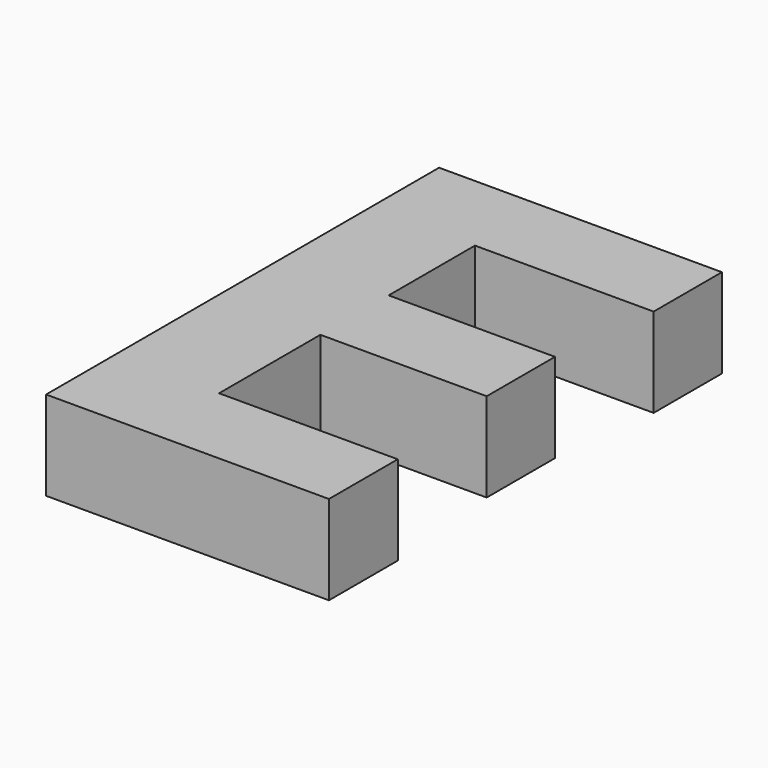
from build123d import *

# Parameters (mm, degrees)
F0_TEXT_SIZE = 77.1269667894
F1_DEPTH     = 10


# Not quite as in the source:
# - Text() gives the source's letters only with a copy of the font that has no kerning and outlines rounded to 1/6400 em; it was checked with that copy


with BuildPart() as f1:
    # F0 (on Top) → F1 (new body)
    with BuildSketch(Plane.XY):
        with Locations((0, 0)):
            Text('E', F0_TEXT_SIZE, font='Open Sans', font_style=FontStyle.BOLD, text_align=(TextAlign.LEFT, TextAlign.BOTTOM))
    extrude(amount=F1_DEPTH)


solid = f1.part
